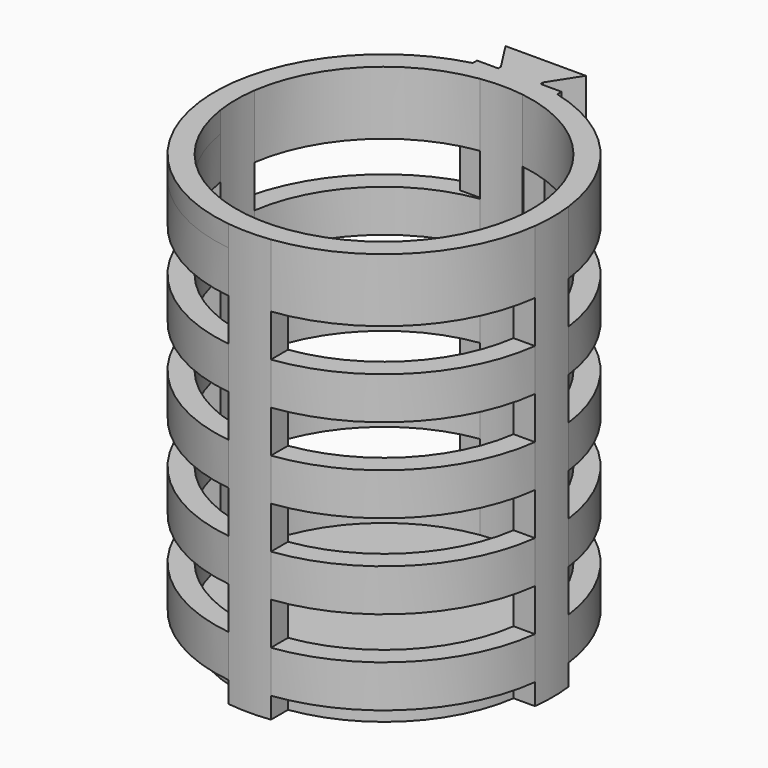
from build123d import *

# Parameters (mm, degrees)
F1_DEPTH = 5
F2_DEPTH = 100
F3_START = 5
F3_DEPTH = 10
F4_START = 25
F4_DEPTH = 10
F5_START = 45
F5_DEPTH = 55
F6_START = 45
F6_DEPTH = 10
F7_START = 65
F7_DEPTH = 10
F8_START = 85
F8_DEPTH = 15


# Not quite as in the source:
# - a pattern or mirror of a feature is missing from the dataset's text; its kind, count and spacing are read off the source's solid


with BuildPart() as f1:
    # F0 (on Top) → F1 (new body)
    with BuildSketch(Plane.XY):
        with BuildLine():
            ThreePointArc((34.6410161514, -5), (34.9101386799, -2.5064351879), (35, 0))
            ThreePointArc((35, 0), (34.9101386799, 2.5064351879), (34.6410161514, 5))
            ThreePointArc((34.6410161514, 5), (24.7487373415, 24.7487373415), (5, 34.6410161514))
            ThreePointArc((5, 34.6410161514), (0, 35), (-5, 34.6410161514))
            ThreePointArc((-5, 34.6410161514), (-24.7487373415, 24.7487373415), (-34.6410161514, 5))
            ThreePointArc((-34.6410161514, 5), (-35, 0), (-34.6410161514, -5))
            ThreePointArc((-34.6410161514, -5), (-24.7487373415, -24.7487373415), (-5, -34.6410161514))
            ThreePointArc((-5, -34.6410161514), (0, -35), (5, -34.6410161514))
            ThreePointArc((5, -34.6410161514), (24.7487373415, -24.7487373415), (34.6410161514, -5))
        make_face()
    extrude(amount=F1_DEPTH)

    # F0 (on Top) → F2 (join)
    with BuildSketch(Plane.XY):
        with BuildLine():
            ThreePointArc((-34.6410161514, -5), (-35, 0), (-34.6410161514, 5))
            Line((-34.6410161514, 5), (-39.686269666, 5))
            ThreePointArc((-39.686269666, 5), (-40, 0), (-39.686269666, -5))
            Line((-39.686269666, -5), (-34.6410161514, -5))
        make_face()
        with BuildLine():
            Line((5, -39.686269666), (5, -34.6410161514))
            ThreePointArc((5, -34.6410161514), (0, -35), (-5, -34.6410161514))
            Line((-5, -34.6410161514), (-5, -39.686269666))
            ThreePointArc((-5, -39.686269666), (0, -40), (5, -39.686269666))
        make_face()
        with BuildLine():
            ThreePointArc((34.6410161514, 5), (34.9101386799, 2.5064351879), (35, 0))
            ThreePointArc((35, 0), (34.9101386799, -2.5064351879), (34.6410161514, -5))
            Line((34.6410161514, -5), (39.686269666, -5))
            ThreePointArc((39.686269666, -5), (40, 0), (39.686269666, 5))
            Line((39.686269666, 5), (34.6410161514, 5))
        make_face()
        with BuildLine():
            ThreePointArc((-5, 34.6410161514), (0, 35), (5, 34.6410161514))
            Line((5, 34.6410161514), (5, 35))
            Line((5, 35), (10, 35))
            Line((10, 35), (10, 38.7298334621))
            Line((10, 38.7298334621), (10, 40))
            Line((10, 40), (5, 40))
            Line((5, 40), (-5, 40))
            Line((-5, 40), (-10, 40))
            Line((-10, 40), (-10, 38.7298334621))
            Line((-10, 38.7298334621), (-10, 35))
            Line((-10, 35), (-5, 35))
            Line((-5, 35), (-5, 34.6410161514))
        make_face()
    extrude(amount=F2_DEPTH)

    # F3_copies: F3 across plane


with BuildPart() as f3:
    # F0 (on Top) → F3 (new body)
    with BuildSketch(Plane.XY.offset(F3_START)):
        with BuildLine():
            Line((-5, -39.686269666), (-5, -34.6410161514))
            ThreePointArc((-5, -34.6410161514), (-24.7487373415, -24.7487373415), (-34.6410161514, -5))
            Line((-34.6410161514, -5), (-39.686269666, -5))
            ThreePointArc((-39.686269666, -5), (-28.2842712475, -28.2842712475), (-5, -39.686269666))
        make_face()
    extrude(amount=F3_DEPTH)


with BuildPart() as f3b:
    # F0 (on Top) → F3, piece 2 (new body)
    with BuildSketch(Plane.XY.offset(F3_START)):
        with BuildLine():
            Line((39.686269666, -5), (34.6410161514, -5))
            ThreePointArc((34.6410161514, -5), (24.7487373415, -24.7487373415), (5, -34.6410161514))
            Line((5, -34.6410161514), (5, -39.686269666))
            ThreePointArc((5, -39.686269666), (28.2842712475, -28.2842712475), (39.686269666, -5))
        make_face()
    extrude(amount=F3_DEPTH)


with BuildPart() as f3c:
    # F0 (on Top) → F3, piece 3 (new body)
    with BuildSketch(Plane.XY.offset(F3_START)):
        with BuildLine():
            ThreePointArc((5, 34.6410161514), (24.7487373415, 24.7487373415), (34.6410161514, 5))
            Line((34.6410161514, 5), (39.686269666, 5))
            ThreePointArc((39.686269666, 5), (30.0267674696, 26.4271306677), (10, 38.7298334621))
            Line((10, 38.7298334621), (10, 35))
            Line((10, 35), (5, 35))
            Line((5, 35), (5, 34.6410161514))
        make_face()
    extrude(amount=F3_DEPTH)


with BuildPart() as f3d:
    # F0 (on Top) → F3, piece 4 (new body)
    with BuildSketch(Plane.XY.offset(F3_START)):
        with BuildLine():
            ThreePointArc((-34.6410161514, 5), (-24.7487373415, 24.7487373415), (-5, 34.6410161514))
            Line((-5, 34.6410161514), (-5, 35))
            Line((-5, 35), (-10, 35))
            Line((-10, 35), (-10, 38.7298334621))
            ThreePointArc((-10, 38.7298334621), (-30.0267674696, 26.4271306677), (-39.686269666, 5))
            Line((-39.686269666, 5), (-34.6410161514, 5))
        make_face()
    extrude(amount=F3_DEPTH)


with BuildPart() as f1_1:
    add(f1.part)
    add(f3.part.mirror(Plane.XY.offset(50)))

    # F0 (on Top) → F4 (join)
    with BuildSketch(Plane.XY.offset(F4_START)):
        with BuildLine():
            Line((-5, -39.686269666), (-5, -34.6410161514))
            ThreePointArc((-5, -34.6410161514), (-24.7487373415, -24.7487373415), (-34.6410161514, -5))
            Line((-34.6410161514, -5), (-39.686269666, -5))
            ThreePointArc((-39.686269666, -5), (-28.2842712475, -28.2842712475), (-5, -39.686269666))
        make_face()
        with BuildLine():
            ThreePointArc((-34.6410161514, 5), (-24.7487373415, 24.7487373415), (-5, 34.6410161514))
            Line((-5, 34.6410161514), (-5, 35))
            Line((-5, 35), (-10, 35))
            Line((-10, 35), (-10, 38.7298334621))
            ThreePointArc((-10, 38.7298334621), (-30.0267674696, 26.4271306677), (-39.686269666, 5))
            Line((-39.686269666, 5), (-34.6410161514, 5))
        make_face()
        with BuildLine():
            ThreePointArc((5, 34.6410161514), (24.7487373415, 24.7487373415), (34.6410161514, 5))
            Line((34.6410161514, 5), (39.686269666, 5))
            ThreePointArc((39.686269666, 5), (30.0267674696, 26.4271306677), (10, 38.7298334621))
            Line((10, 38.7298334621), (10, 35))
            Line((10, 35), (5, 35))
            Line((5, 35), (5, 34.6410161514))
        make_face()
        with BuildLine():
            Line((39.686269666, -5), (34.6410161514, -5))
            ThreePointArc((34.6410161514, -5), (24.7487373415, -24.7487373415), (5, -34.6410161514))
            Line((5, -34.6410161514), (5, -39.686269666))
            ThreePointArc((5, -39.686269666), (28.2842712475, -28.2842712475), (39.686269666, -5))
        make_face()
    extrude(amount=F4_DEPTH)

    # F0 (on Top) → F5 (join)
    with BuildSketch(Plane.XY.offset(F5_START)):
        Polygon((-5, 40), (5, 40), (5, 40.8), (9.5, 47.8), (-9.5, 47.8), (-5, 40.8), align=None)
    extrude(amount=F5_DEPTH)

    # F0 (on Top) → F6 (join)
    with BuildSketch(Plane.XY.offset(F6_START)):
        with BuildLine():
            ThreePointArc((-34.6410161514, 5), (-24.7487373415, 24.7487373415), (-5, 34.6410161514))
            Line((-5, 34.6410161514), (-5, 35))
            Line((-5, 35), (-10, 35))
            Line((-10, 35), (-10, 38.7298334621))
            ThreePointArc((-10, 38.7298334621), (-30.0267674696, 26.4271306677), (-39.686269666, 5))
            Line((-39.686269666, 5), (-34.6410161514, 5))
        make_face()
        with BuildLine():
            Line((-5, -39.686269666), (-5, -34.6410161514))
            ThreePointArc((-5, -34.6410161514), (-24.7487373415, -24.7487373415), (-34.6410161514, -5))
            Line((-34.6410161514, -5), (-39.686269666, -5))
            ThreePointArc((-39.686269666, -5), (-28.2842712475, -28.2842712475), (-5, -39.686269666))
        make_face()
        with BuildLine():
            Line((39.686269666, -5), (34.6410161514, -5))
            ThreePointArc((34.6410161514, -5), (24.7487373415, -24.7487373415), (5, -34.6410161514))
            Line((5, -34.6410161514), (5, -39.686269666))
            ThreePointArc((5, -39.686269666), (28.2842712475, -28.2842712475), (39.686269666, -5))
        make_face()
        with BuildLine():
            ThreePointArc((5, 34.6410161514), (24.7487373415, 24.7487373415), (34.6410161514, 5))
            Line((34.6410161514, 5), (39.686269666, 5))
            ThreePointArc((39.686269666, 5), (30.0267674696, 26.4271306677), (10, 38.7298334621))
            Line((10, 38.7298334621), (10, 35))
            Line((10, 35), (5, 35))
            Line((5, 35), (5, 34.6410161514))
        make_face()
    extrude(amount=F6_DEPTH)

    # F0 (on Top) → F7 (join)
    with BuildSketch(Plane.XY.offset(F7_START)):
        with BuildLine():
            Line((39.686269666, -5), (34.6410161514, -5))
            ThreePointArc((34.6410161514, -5), (24.7487373415, -24.7487373415), (5, -34.6410161514))
            Line((5, -34.6410161514), (5, -39.686269666))
            ThreePointArc((5, -39.686269666), (28.2842712475, -28.2842712475), (39.686269666, -5))
        make_face()
        with BuildLine():
            Line((-5, -39.686269666), (-5, -34.6410161514))
            ThreePointArc((-5, -34.6410161514), (-24.7487373415, -24.7487373415), (-34.6410161514, -5))
            Line((-34.6410161514, -5), (-39.686269666, -5))
            ThreePointArc((-39.686269666, -5), (-28.2842712475, -28.2842712475), (-5, -39.686269666))
        make_face()
        with BuildLine():
            ThreePointArc((-34.6410161514, 5), (-24.7487373415, 24.7487373415), (-5, 34.6410161514))
            Line((-5, 34.6410161514), (-5, 35))
            Line((-5, 35), (-10, 35))
            Line((-10, 35), (-10, 38.7298334621))
            ThreePointArc((-10, 38.7298334621), (-30.0267674696, 26.4271306677), (-39.686269666, 5))
            Line((-39.686269666, 5), (-34.6410161514, 5))
        make_face()
        with BuildLine():
            ThreePointArc((5, 34.6410161514), (24.7487373415, 24.7487373415), (34.6410161514, 5))
            Line((34.6410161514, 5), (39.686269666, 5))
            ThreePointArc((39.686269666, 5), (30.0267674696, 26.4271306677), (10, 38.7298334621))
            Line((10, 38.7298334621), (10, 35))
            Line((10, 35), (5, 35))
            Line((5, 35), (5, 34.6410161514))
        make_face()
    extrude(amount=F7_DEPTH)

    # F0 (on Top) → F8 (join)
    with BuildSketch(Plane.XY.offset(F8_START)):
        with BuildLine():
            Line((39.686269666, -5), (34.6410161514, -5))
            ThreePointArc((34.6410161514, -5), (24.7487373415, -24.7487373415), (5, -34.6410161514))
            Line((5, -34.6410161514), (5, -39.686269666))
            ThreePointArc((5, -39.686269666), (28.2842712475, -28.2842712475), (39.686269666, -5))
        make_face()
        with BuildLine():
            Line((-5, -39.686269666), (-5, -34.6410161514))
            ThreePointArc((-5, -34.6410161514), (-24.7487373415, -24.7487373415), (-34.6410161514, -5))
            Line((-34.6410161514, -5), (-39.686269666, -5))
            ThreePointArc((-39.686269666, -5), (-28.2842712475, -28.2842712475), (-5, -39.686269666))
        make_face()
        with BuildLine():
            ThreePointArc((-34.6410161514, 5), (-24.7487373415, 24.7487373415), (-5, 34.6410161514))
            Line((-5, 34.6410161514), (-5, 35))
            Line((-5, 35), (-10, 35))
            Line((-10, 35), (-10, 38.7298334621))
            ThreePointArc((-10, 38.7298334621), (-30.0267674696, 26.4271306677), (-39.686269666, 5))
            Line((-39.686269666, 5), (-34.6410161514, 5))
        make_face()
        with BuildLine():
            ThreePointArc((5, 34.6410161514), (24.7487373415, 24.7487373415), (34.6410161514, 5))
            Line((34.6410161514, 5), (39.686269666, 5))
            ThreePointArc((39.686269666, 5), (30.0267674696, 26.4271306677), (10, 38.7298334621))
            Line((10, 38.7298334621), (10, 35))
            Line((10, 35), (5, 35))
            Line((5, 35), (5, 34.6410161514))
        make_face()
    extrude(amount=F8_DEPTH)


solid = Compound([f3.part, f3b.part, f3c.part, f3d.part, f1_1.part])
